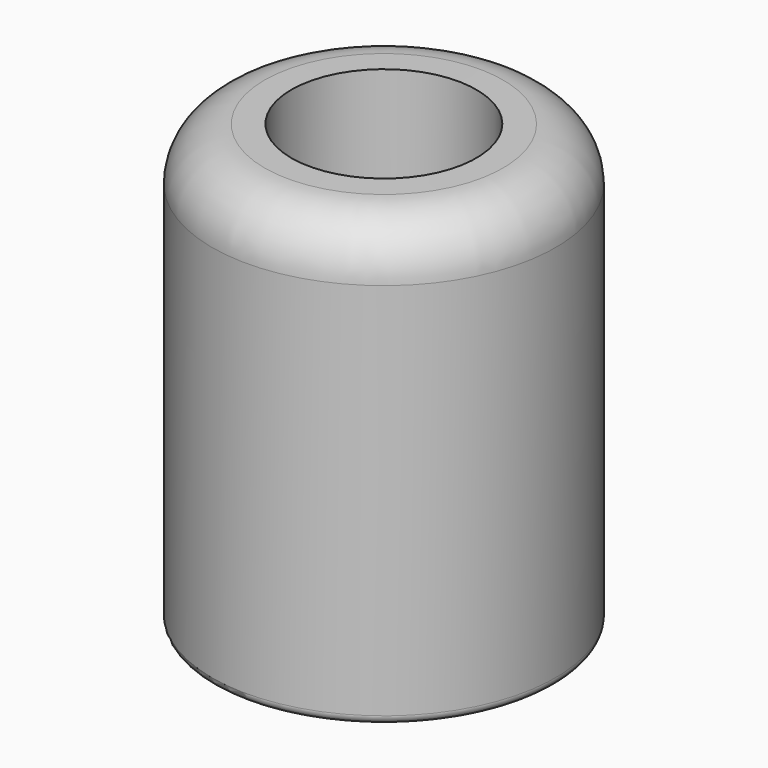
from build123d import *

# Parameters (mm, degrees)
F2_R = 0.99999
F3_R = 2


# Not quite as in the source:
# - a fillet or chamfer is up to 0.001 mm smaller than in the source, because OpenCascade refuses the exact size


with BuildPart() as f1:
    # F0 (on Front) → F1 (revolve)
    with BuildSketch(Plane.XZ):
        with BuildLine():
            Line((-10.5, 0), (-10.5, 30))
            Line((-10.5, 30), (-13.532049904, 29.9838036175))
            ThreePointArc((-13.532049904, 29.9838036175), (-17.7539569476, 28.2151833802), (-19.5, 23.9838892179))
            Line((-19.5, 23.9838892179), (-19.5, 20))
            Line((-19.5, 20), (-19.5, -20))
            Line((-19.5, -20), (-17.5, -20))
            Line((-17.5, -20), (-17.5, 20))
            Line((-17.5, 20), (-15.5, 20))
            Line((-15.5, 20), (-15.5, 0))
            Line((-15.5, 0), (-10.5, 0))
        make_face()
    revolve(axis=Axis((0, 0, 11.9062974118), (0, 0, -1)))

    # F2 (radius 1 in the source; OpenCascade refuses exactly that, so slightly less here)
    f2_edges = [f1.edges().sort_by_distance(p)[0] for p in [
        (17.5, 0, -20),
        (19.5, 0, -20),
    ]]
    fillet(f2_edges, radius=F2_R)

    # F3
    f3_edges = [f1.edges().sort_by_distance(p)[0] for p in [
        (10.5, 0, 0),
        (15.5, 0, 0),
    ]]
    fillet(f3_edges, radius=F3_R)


solid = f1.part
